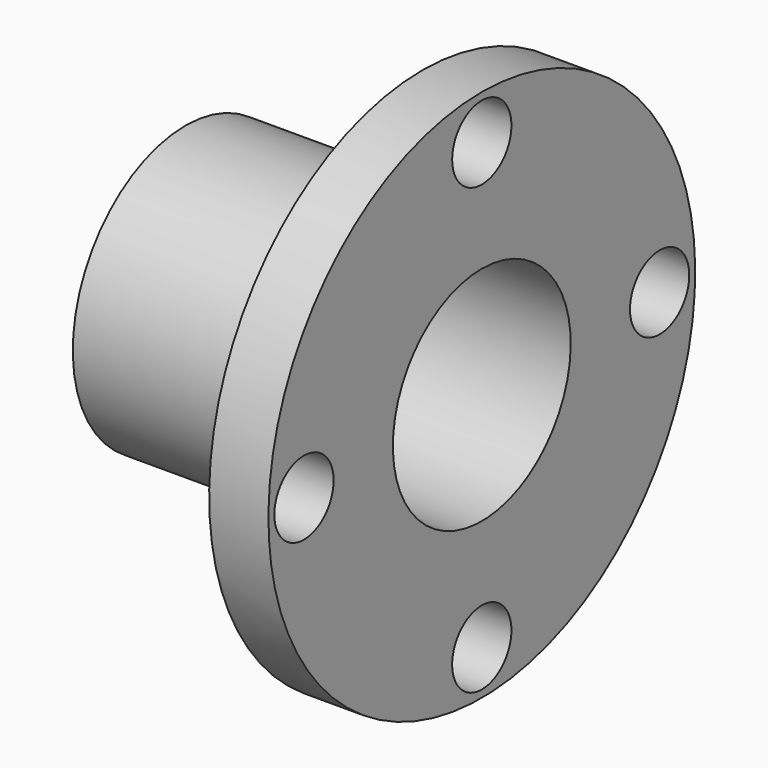
from build123d import *

# Parameters (mm, degrees)
F2_R            = 12.5
F3_DEPTH        = 20.001
F3_COPIES_COUNT = 4


# Not quite as in the source:
# - a pattern or mirror of a feature is missing from the dataset's text; its kind, count and spacing are read off the source's solid


with BuildPart() as f1:
    # F0 (on Front) → F1 (revolve)
    with BuildSketch(Plane.XZ):
        Polygon((-100, 37.5), (0, 37.5), (0, 90), (-20, 90), (-20, 47.5), (-100, 47.5), align=None)
    revolve(axis=Axis((-90.7405540347, 0, 0), (-1, 0, 0)))

    # F2 (on face) → F3 (cut, through all)
    with BuildSketch(Plane(origin=(-20, 0, 0), x_dir=(0, -1, 0), z_dir=(-1, 0, 0))):
        with Locations((0, 75)):
            Circle(F2_R)
    f3 = extrude(amount=-F3_DEPTH, mode=Mode.SUBTRACT)

    # F3_copies: F3 ×4 about axis
    f3_copies_axis = Axis((0, 0, 0), (1, 0, 0))
    for i in range(1, F3_COPIES_COUNT):
        add(f3.rotate(f3_copies_axis, i * 360 / F3_COPIES_COUNT), mode=Mode.SUBTRACT)


solid = f1.part
